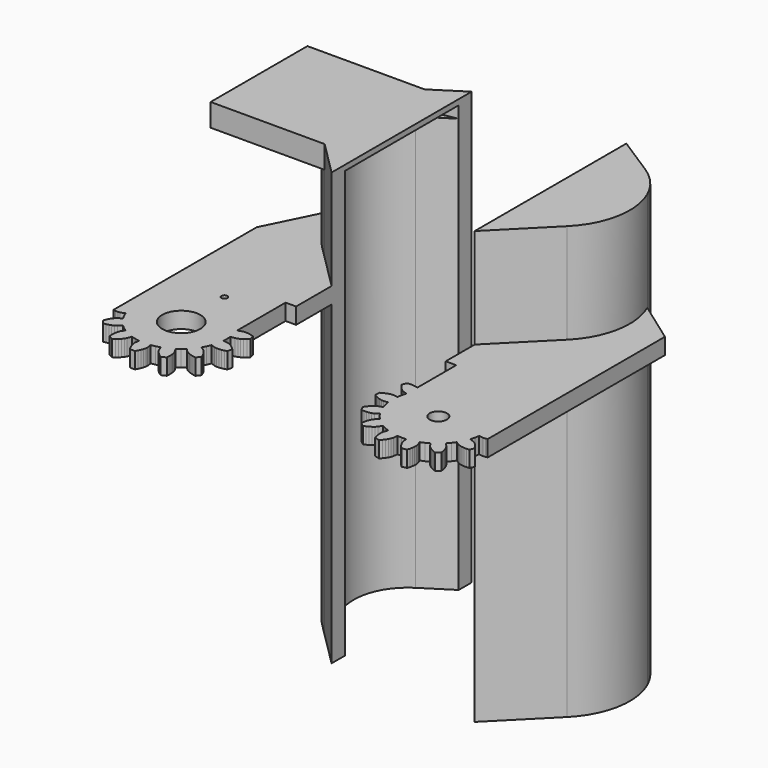
from build123d import *

# Parameters (mm, degrees)
F1_DEPTH  = 1.5
F0_R      = 1.6
F2_DEPTH  = 20
F3_DEPTH  = 60
F4_DEPTH  = 19
F5_DEPTH  = 16.8
F6_DEPTH  = 16.8
F7_DEPTH  = 15.8
F8_DEPTH  = 19
F9_DEPTH  = 15.8
F10_DEPTH = 1.5


# Not quite as in the source:
# - ends of sketch curves that miss each other by under 0.0002 mm in the source are joined


with BuildPart() as f1:
    # F0 (on Top) → F1 (new body, symmetric)
    with BuildSketch(Plane.XY):
        Polygon((-12.6828804, -37.9996929195), (-11.8884367355, -38.2222305677), (-11.8880267366, -38.2224279172), (-11.075543, -38.3664943195), (-11.1792258, -39.1773131195), (-11.1500412, -39.5862277195), (-11.049381, -40.0020257195), (-10.8967016, -40.4206431195), (-10.6978958, -40.8390065195), (-10.4565196, -41.2543727195), (-9.5434404, -41.2543727195), (-9.302115, -40.8390065195), (-9.1033092, -40.4206431195), (-8.950579, -40.0020257195), (-8.8499188, -39.5862277195), (-8.820785, -39.1773131195), (-8.9244678, -38.3664943195), (-8.1119840634, -38.2224279172), (-8.1115408, -38.2223493195), (-7.3171558, -37.9996929195), (-7.0589394, -38.7751549195), (-6.8550028, -39.1308311195), (-6.5838324, -39.4619201195), (-6.2647068, -39.7727145195), (-5.9041792, -40.0633667195), (-5.5066184, -40.3329369195), (-4.6838108, -39.9365445195), (-4.646549, -39.4578053195), (-4.6491144, -38.9947125195), (-4.693031, -38.5513555195), (-4.7828454, -38.1327635195), (-4.9339246, -37.7516365195), (-5.3789072, -37.0664715195), (-4.7096916266, -36.5840362135), (-4.709287, -36.5837445195), (-4.0899842, -36.0385589195), (-3.5209988, -36.6249941195), (-3.1831534, -36.8570993195), (-2.7948636, -37.0377695195), (-2.3725632, -37.1791713195), (-1.9218148, -37.2846829195), (-1.4464538, -37.3550663195), (-0.8770112, -36.6409453195), (-1.0512806, -36.1933973195), (-1.2544552, -35.7773199195), (-1.4865096, -35.3969041195), (-1.7489424, -35.0588555195), (-2.0504658, -34.7809287195), (-2.7488388, -34.3565455195), (-2.3551745142, -33.6315615111), (-2.3549356, -33.6311215195), (-2.0336002, -32.8714075195), (-1.2662154, -33.1527887195), (-0.86106, -33.2152727195), (-0.4331716, -33.2096847195), (0.0087884, -33.1539317195), (0.4607052, -33.0533223195), (0.9195562, -32.9104727195), (1.1227562, -32.0200757195), (0.7714742, -31.6924411195), (0.4079494, -31.4057259195), (0.033782, -31.1636639195), (-0.3494024, -30.9728083195), (-0.741426, -30.8533775195), (-1.5548356, -30.7739771195), (-1.5148031909, -29.9499745831), (-1.5147798, -29.9494931195), (-1.5548356, -29.1254663195), (-0.741426, -29.0460913195), (-0.3494024, -28.9266605195), (0.033782, -28.7358049195), (0.4079494, -28.4937683195), (0.7714742, -28.2070531195), (1.1227562, -27.8793931195), (0.9195562, -26.9889961195), (0.4607052, -26.8461465195), (0.0087884, -26.7455371195), (-0.4331716, -26.6898095195), (-0.86106, -26.6842215195), (-1.2662154, -26.7467055195), (-1.999996, -27.0157423195), (-1.999996, -15.8072914928), (-0.05, -15.8072914928), (-0.05, -8.999886363), (-7.8088611939, -1.2753778), (-20.002250767, -1.2753778), (-20.0087992, -33.1539317195), (-19.5667884, -33.2096847195), (-19.1389, -33.2152727195), (-18.7337954, -33.1527887195), (-17.9664106, -32.8714075195), (-17.6450069939, -33.6311141557), (-17.6448212, -33.6315533195), (-17.251172, -34.3565455195), (-17.9495196, -34.7809287195), (-18.2510684, -35.0588555195), (-18.5134504, -35.3969041195), (-18.745581, -35.7773199195), (-18.9487302, -36.1933973195), (-19.1229996, -36.6409453195), (-18.5535062, -37.3550663195), (-18.078196, -37.2846829195), (-17.6274476, -37.1791713195), (-17.2051218, -37.0377695195), (-16.8168066, -36.8570993195), (-16.479012, -36.6249941195), (-15.9100012, -36.0385589195), (-15.2906723648, -36.583686083), (-15.2903174, -36.5839985195), (-14.6211036, -37.0664715195), (-15.0660862, -37.7516365195), (-15.2171654, -38.1327635195), (-15.306929, -38.5513555195), (-15.3509218, -38.9947125195), (-15.3534618, -39.4578053195), (-15.3162, -39.9365445195), (-14.493367, -40.3329369195), (-14.0958062, -40.0633667195), (-13.735304, -39.7727145195), (-13.4161784, -39.4619201195), (-13.1449572, -39.1308311195), (-12.9410968, -38.7751549195), align=None)
        with BuildLine():
            ThreePointArc((-9.99998, -26.4247471195), (-7.5074285963, -27.4571957159), (-6.47498, -29.9497471195))
            ThreePointArc((-6.47498, -29.9497471195), (-12.4925314037, -32.4422985232), (-9.99998, -26.4247471195))
        make_face(mode=Mode.SUBTRACT)
        with BuildLine():
            ThreePointArc((-9.4549722, -19.9497471195), (-9.6146012888, -20.3351258307), (-9.99998, -20.4947549195))
            ThreePointArc((-9.99998, -20.4947549195), (-10.3853587112, -19.5643684084), (-9.4549722, -19.9497471195))
        make_face(mode=Mode.SUBTRACT)
        Polygon((-6.3914999282, -1.2753778), (-7.8088611939, -1.2753778), (-0.05, -8.999886363), (-0.05, -7.5888005143), align=None)
        Polygon((-8.4115295291, -0.6753778), (-7.8088611939, -1.2753778), (-6.3914999282, -1.2753778), (-6.9941682635, -0.6753778), align=None)
        with BuildLine():
            Line((-20.0019887813, 0), (-20.0021275162, -0.6753778))
            Line((-20.0021275162, -0.6753778), (-8.4115295291, -0.6753778))
            Line((-8.4115295291, -0.6753778), (-6.9941682635, -0.6753778))
            Line((-6.9941682635, -0.6753778), (-8.8192027426, 1.1415762748))
            ThreePointArc((-8.8192027426, 1.1415762748), (-11.5431807788, 5.203648739), (-12.5000003164, 10))
            Line((-12.5000003164, 10), (-15.0591228454, 10))
            Line((-15.0591228454, 10), (-20.0019887813, 0))
        make_face()
        with BuildLine():
            Line((-12.1022985118, 15.9820039061), (-15.0591228454, 10))
            Line((-15.0591228454, 10), (-12.5000003164, 10))
            ThreePointArc((-12.5000003164, 10), (-11.8911847625, 13.8535351113), (-10.1240431199, 17.331695494))
            Line((-10.1240431199, 17.331695494), (-12.1022985118, 15.9820039061))
        make_face()
        Polygon((-20.0021275162, -0.6753778), (-20.002250767, -1.2753778), (-7.8088611939, -1.2753778), (-8.4115295291, -0.6753778), align=None)
    extrude(amount=F1_DEPTH, both=True)



with BuildPart() as f1b:
    # F0 (on Top) → F1, piece 2 (new body, symmetric)
    with BuildSketch(Plane.XY):
        with BuildLine():
            Line((45.5568809356, -32.5242657195), (45.7794119864, -31.729845607))
            Line((45.7794119864, -31.729845607), (45.7796203111, -31.7294128346))
            Line((45.7796203111, -31.7294128346), (45.9237077356, -30.9169283195))
            Line((45.9237077356, -30.9169283195), (46.7345011356, -31.0206111195))
            Line((46.7345011356, -31.0206111195), (47.1434157356, -30.9914519195))
            Line((47.1434157356, -30.9914519195), (47.5068643356, -30.9034663195))
            Line((47.5068643356, -30.9034663195), (47.5068643356, 10.1083564))
            Line((47.5068643356, 10.1083564), (39.8461772472, 15.5849402666))
            ThreePointArc((39.8461772472, 15.5849402666), (40.7766908436, 7.6257287323), (37.0316684565, 0.541259019))
            Line((37.0316684565, 0.541259019), (27.5569297356, -8.9911811067))
            Line((27.5569297356, -8.9911811067), (27.5569297356, -15.6989350928))
            Line((27.5569297356, -15.6989350928), (29.5069257356, -15.6989350928))
            Line((29.5069257356, -15.6989350928), (29.5069257356, -24.6967985195))
            Line((29.5069257356, -24.6967985195), (29.3238933356, -24.6242561195))
            Line((29.3238933356, -24.6242561195), (28.9053267356, -24.5344163195))
            Line((28.9053267356, -24.5344163195), (28.4619443356, -24.4904997195))
            Line((28.4619443356, -24.4904997195), (27.9988769356, -24.4879343195))
            Line((27.9988769356, -24.4879343195), (27.5201123356, -24.5252215195))
            Line((27.5201123356, -24.5252215195), (27.1237453356, -25.3480037195))
            Line((27.1237453356, -25.3480037195), (27.3933155356, -25.7455645195))
            Line((27.3933155356, -25.7455645195), (27.6839931356, -26.1060921195))
            Line((27.6839931356, -26.1060921195), (27.9947367356, -26.4252177195))
            Line((27.9947367356, -26.4252177195), (28.3259019356, -26.6964135195))
            Line((28.3259019356, -26.6964135195), (28.6815781356, -26.9003247195))
            Line((28.6815781356, -26.9003247195), (29.4569385356, -27.1585411195))
            Line((29.4569385356, -27.1585411195), (29.2345090358, -27.9529612023))
            Line((29.2345090358, -27.9529612023), (29.2343837356, -27.9534087195))
            Line((29.2343837356, -27.9534087195), (29.0901625356, -28.7658785195))
            Line((29.0901625356, -28.7658785195), (28.2793183356, -28.6621957195))
            Line((28.2793183356, -28.6621957195), (27.8704545356, -28.6913041195))
            Line((27.8704545356, -28.6913041195), (27.4546819356, -28.7919643195))
            Line((27.4546819356, -28.7919643195), (27.0360137356, -28.9447199195))
            Line((27.0360137356, -28.9447199195), (26.6177011356, -29.1435003195))
            Line((26.6177011356, -29.1435003195), (26.2023095356, -29.3848257195))
            Line((26.2023095356, -29.3848257195), (26.2023095356, -30.2979303195))
            Line((26.2023095356, -30.2979303195), (26.6177011356, -30.5392811195))
            Line((26.6177011356, -30.5392811195), (27.0360137356, -30.7380869195))
            Line((27.0360137356, -30.7380869195), (27.4546819356, -30.8907917195))
            Line((27.4546819356, -30.8907917195), (27.8704545356, -30.9914519195))
            Line((27.8704545356, -30.9914519195), (28.2793183356, -31.0206111195))
            Line((28.2793183356, -31.0206111195), (29.0901625356, -30.9169283195))
            Line((29.0901625356, -30.9169283195), (29.2343007326, -31.7294128446))
            Line((29.2343007326, -31.7294128446), (29.2343837356, -31.7298807195))
            Line((29.2343837356, -31.7298807195), (29.4569385356, -32.5242657195))
            Line((29.4569385356, -32.5242657195), (28.6815781356, -32.7824821195))
            Line((28.6815781356, -32.7824821195), (28.3259019356, -32.9863679195))
            Line((28.3259019356, -32.9863679195), (27.9947367356, -33.2575891195))
            Line((27.9947367356, -33.2575891195), (27.6839931356, -33.5766893195))
            Line((27.6839931356, -33.5766893195), (27.3933155356, -33.9371915195))
            Line((27.3933155356, -33.9371915195), (27.1237453356, -34.3347523195))
            Line((27.1237453356, -34.3347523195), (27.5201123356, -35.1575853195))
            Line((27.5201123356, -35.1575853195), (27.9988769356, -35.1948725195))
            Line((27.9988769356, -35.1948725195), (28.4619443356, -35.1923071195))
            Line((28.4619443356, -35.1923071195), (28.9053267356, -35.1483397195))
            Line((28.9053267356, -35.1483397195), (29.3238933356, -35.0585507195))
            Line((29.3238933356, -35.0585507195), (29.7050457356, -34.9074715195))
            Line((29.7050457356, -34.9074715195), (30.3902107356, -34.4624889195))
            Line((30.3902107356, -34.4624889195), (30.8726460484, -35.1317298871))
            Line((30.8726460484, -35.1317298871), (30.8729377356, -35.1321345195))
            Line((30.8729377356, -35.1321345195), (31.4180979356, -35.7513865195))
            Line((31.4180979356, -35.7513865195), (30.8316881356, -36.3203973195))
            Line((30.8316881356, -36.3203973195), (30.5995829356, -36.6582173195))
            Line((30.5995829356, -36.6582173195), (30.4189127356, -37.0465071195))
            Line((30.4189127356, -37.0465071195), (30.2775109356, -37.4688583195))
            Line((30.2775109356, -37.4688583195), (30.1719993356, -37.9196067195))
            Line((30.1719993356, -37.9196067195), (30.1016159356, -38.3949169195))
            Line((30.1016159356, -38.3949169195), (30.8157369356, -38.9643849195))
            Line((30.8157369356, -38.9643849195), (31.2632849356, -38.7901155195))
            Line((31.2632849356, -38.7901155195), (31.6793623356, -38.5869663195))
            Line((31.6793623356, -38.5869663195), (32.0597527356, -38.3548611195))
            Line((32.0597527356, -38.3548611195), (32.3978267356, -38.0924537195))
            Line((32.3978267356, -38.0924537195), (32.6757535356, -37.7909049195))
            Line((32.6757535356, -37.7909049195), (33.1001367356, -37.0925827195))
            Line((33.1001367356, -37.0925827195), (33.8251420267, -37.4861824058))
            Line((33.8251420267, -37.4861824058), (33.8255607356, -37.4864097195))
            Line((33.8255607356, -37.4864097195), (34.5852747356, -37.8077959195))
            Line((34.5852747356, -37.8077959195), (34.3038935356, -38.5752061195))
            Line((34.3038935356, -38.5752061195), (34.2414095356, -38.9803107195))
            Line((34.2414095356, -38.9803107195), (34.2469975356, -39.4081737195))
            Line((34.2469975356, -39.4081737195), (34.3027505356, -39.8501845195))
            Line((34.3027505356, -39.8501845195), (34.4033599356, -40.3021267195))
            Line((34.4033599356, -40.3021267195), (34.5461841356, -40.7609777195))
            Line((34.5461841356, -40.7609777195), (35.4366065356, -40.9641777195))
            Line((35.4366065356, -40.9641777195), (35.7642411356, -40.6128957195))
            Line((35.7642411356, -40.6128957195), (36.0509563356, -40.2493201195))
            Line((36.0509563356, -40.2493201195), (36.2929929356, -39.8751781195))
            Line((36.2929929356, -39.8751781195), (36.4838739356, -39.4919429195))
            Line((36.4838739356, -39.4919429195), (36.6033047356, -39.0999955195))
            Line((36.6033047356, -39.0999955195), (36.6826797356, -38.2865605195))
            Line((36.6826797356, -38.2865605195), (37.5067076121, -38.3265941598))
            Line((37.5067076121, -38.3265941598), (37.5071637356, -38.3266163195))
            Line((37.5071637356, -38.3266163195), (38.3311651356, -38.2865605195))
            Line((38.3311651356, -38.2865605195), (38.4105909356, -39.0999955195))
            Line((38.4105909356, -39.0999955195), (38.5299963356, -39.4919429195))
            Line((38.5299963356, -39.4919429195), (38.7208773356, -39.8751781195))
            Line((38.7208773356, -39.8751781195), (38.9629139356, -40.2493201195))
            Line((38.9629139356, -40.2493201195), (39.2496291356, -40.6128957195))
            Line((39.2496291356, -40.6128957195), (39.5772891356, -40.9641777195))
            Line((39.5772891356, -40.9641777195), (40.4676861356, -40.7609777195))
            Line((40.4676861356, -40.7609777195), (40.6105103356, -40.3021267195))
            Line((40.6105103356, -40.3021267195), (40.7111451356, -39.8501845195))
            Line((40.7111451356, -39.8501845195), (40.7668727356, -39.4081737195))
            Line((40.7668727356, -39.4081737195), (40.7724607356, -38.9803107195))
            Line((40.7724607356, -38.9803107195), (40.7099767356, -38.5752061195))
            Line((40.7099767356, -38.5752061195), (40.4285955356, -37.8077959195))
            Line((40.4285955356, -37.8077959195), (41.1883021717, -37.4863923134))
            Line((41.1883021717, -37.4863923134), (41.1887413356, -37.4862065195))
            Line((41.1887413356, -37.4862065195), (41.9137335356, -37.0925827195))
            Line((41.9137335356, -37.0925827195), (42.3381421356, -37.7909049195))
            Line((42.3381421356, -37.7909049195), (42.6160435356, -38.0924537195))
            Line((42.6160435356, -38.0924537195), (42.9541175356, -38.3548611195))
            Line((42.9541175356, -38.3548611195), (43.3345079356, -38.5869663195))
            Line((43.3345079356, -38.5869663195), (43.7505853356, -38.7901155195))
            Line((43.7505853356, -38.7901155195), (44.1981333356, -38.9643849195))
            Line((44.1981333356, -38.9643849195), (44.9122543356, -38.3949169195))
            Line((44.9122543356, -38.3949169195), (44.8418709356, -37.9196067195))
            Line((44.8418709356, -37.9196067195), (44.7363593356, -37.4688583195))
            Line((44.7363593356, -37.4688583195), (44.5949575356, -37.0465071195))
            Line((44.5949575356, -37.0465071195), (44.4142873356, -36.6582173195))
            Line((44.4142873356, -36.6582173195), (44.1821821356, -36.3203973195))
            Line((44.1821821356, -36.3203973195), (43.5957723356, -35.7513865195))
            Line((43.5957723356, -35.7513865195), (44.1408615089, -35.1320720054))
            Line((44.1408615089, -35.1320720054), (44.1411865356, -35.1317027195))
            Line((44.1411865356, -35.1317027195), (44.6236595356, -34.4624889195))
            Line((44.6236595356, -34.4624889195), (45.3088245356, -34.9074715195))
            Line((45.3088245356, -34.9074715195), (45.6899769356, -35.0585507195))
            Line((45.6899769356, -35.0585507195), (46.1085435356, -35.1483397195))
            Line((46.1085435356, -35.1483397195), (46.5519259356, -35.1923071195))
            Line((46.5519259356, -35.1923071195), (47.0149933356, -35.1948725195))
            Line((47.0149933356, -35.1948725195), (47.4937325356, -35.1575853195))
            Line((47.4937325356, -35.1575853195), (47.8901249356, -34.3347523195))
            Line((47.8901249356, -34.3347523195), (47.6205547356, -33.9371915195))
            Line((47.6205547356, -33.9371915195), (47.3299025356, -33.5766893195))
            Line((47.3299025356, -33.5766893195), (47.0191335356, -33.2575891195))
            Line((47.0191335356, -33.2575891195), (46.6880191356, -32.9863679195))
            Line((46.6880191356, -32.9863679195), (46.3323429356, -32.7824821195))
            Line((46.3323429356, -32.7824821195), (45.5568809356, -32.5242657195))
        make_face()
        with Locations((37.5069097356, -29.8413907195)):
            Circle(F0_R, mode=Mode.SUBTRACT)
    extrude(amount=F1_DEPTH, both=True)



with BuildPart() as f2:
    # F0 (on Top) → F2 (new body)
    with BuildSketch(Plane.XY):
        with BuildLine():
            Line((-8.8192027426, 1.1415762748), (-6.9941682635, -0.6753778))
            Line((-6.9941682635, -0.6753778), (-0.05, -4.5405198881))
            Line((-0.05, -4.5405198881), (-7.28327834, 3.1477115777))
            ThreePointArc((-7.28327834, 3.1477115777), (-9.9219987158, 11.2465718924), (-5.3618740808, 18.4409896542))
            Line((-5.3618740808, 18.4409896542), (-0.05, 21.8151911543))
            Line((-0.05, 21.8151911543), (-6.7420944452, 20.5258809799))
            ThreePointArc((-6.7420944452, 20.5258809799), (-8.5829688524, 19.0874998536), (-10.1240431199, 17.331695494))
            ThreePointArc((-10.1240431199, 17.331695494), (-11.8911847625, 13.8535351113), (-12.5000003164, 10))
            ThreePointArc((-12.5000003164, 10), (-11.5431807788, 5.203648739), (-8.8192027426, 1.1415762748))
        make_face()
        Polygon((-5.8053634872, 21.1258809799), (-6.7420944452, 20.5258809799), (-0.05, 21.8151911543), (-0.05, 22.999886363), (-0.05, 24.8123376548), align=None)
        Polygon((-6.9941682635, -0.6753778), (-6.3914999282, -1.2753778), (-0.05, -7.5888005143), (-0.05, -5.999886363), (-0.05, -4.5405198881), align=None)
        with BuildLine():
            Line((-7.28327834, 3.1477115777), (-0.05, -4.5405198881))
            Line((-0.05, -4.5405198881), (-0.05, 21.8151911543))
            Line((-0.05, 21.8151911543), (-5.3618740808, 18.4409896542))
            ThreePointArc((-5.3618740808, 18.4409896542), (-9.9219987158, 11.2465718924), (-7.28327834, 3.1477115777))
        make_face()
        with BuildLine():
            ThreePointArc((-17.0059758203, 20.5258809799), (-19.2368888885, 15.4716989952), (-19.9999346, 10))
            Line((-19.9999346, 10), (-15.0591228454, 10))
            Line((-15.0591228454, 10), (-12.1022985118, 15.9820039061))
            Line((-12.1022985118, 15.9820039061), (-10.1240431199, 17.331695494))
            ThreePointArc((-10.1240431199, 17.331695494), (-8.5829688524, 19.0874998536), (-6.7420944452, 20.5258809799))
            Line((-6.7420944452, 20.5258809799), (-17.0059758203, 20.5258809799))
        make_face()
        with BuildLine():
            Line((-27.5000003164, 10), (-19.9999346, 10))
            ThreePointArc((-19.9999346, 10), (-19.2368888885, 15.4716989952), (-17.0059758203, 20.5258809799))
            Line((-17.0059758203, 20.5258809799), (-27.5000003164, 20.5258809799))
            Line((-27.5000003164, 20.5258809799), (-27.5000003164, 10))
        make_face()
        Polygon((-27.5000003164, -0.6753778), (-20.0021275162, -0.6753778), (-20.0019887813, 0), (-19.9999346, 10), (-27.5000003164, 10), align=None)
        Polygon((-19.9999346, 10), (-20.0019887813, 0), (-15.0591228454, 10), align=None)
        with BuildLine():
            Line((-20.0019887813, 0), (-20.0021275162, -0.6753778))
            Line((-20.0021275162, -0.6753778), (-8.4115295291, -0.6753778))
            Line((-8.4115295291, -0.6753778), (-6.9941682635, -0.6753778))
            Line((-6.9941682635, -0.6753778), (-8.8192027426, 1.1415762748))
            ThreePointArc((-8.8192027426, 1.1415762748), (-11.5431807788, 5.203648739), (-12.5000003164, 10))
            Line((-12.5000003164, 10), (-15.0591228454, 10))
            Line((-15.0591228454, 10), (-20.0019887813, 0))
        make_face()
        with BuildLine():
            Line((-12.1022985118, 15.9820039061), (-15.0591228454, 10))
            Line((-15.0591228454, 10), (-12.5000003164, 10))
            ThreePointArc((-12.5000003164, 10), (-11.8911847625, 13.8535351113), (-10.1240431199, 17.331695494))
            Line((-10.1240431199, 17.331695494), (-12.1022985118, 15.9820039061))
        make_face()
        with BuildLine():
            ThreePointArc((-16.6196316573, 21.1258809799), (-16.8154800574, 20.82760428), (-17.0059758203, 20.5258809799))
            Line((-17.0059758203, 20.5258809799), (-6.7420944452, 20.5258809799))
            Line((-6.7420944452, 20.5258809799), (-5.8053634872, 21.1258809799))
            Line((-5.8053634872, 21.1258809799), (-16.6196316573, 21.1258809799))
        make_face()
        with BuildLine():
            Line((-27.5000003164, 20.5258809799), (-17.0059758203, 20.5258809799))
            ThreePointArc((-17.0059758203, 20.5258809799), (-16.8154800574, 20.82760428), (-16.6196316573, 21.1258809799))
            Line((-16.6196316573, 21.1258809799), (-27.5000003164, 21.1258809799))
            Line((-27.5000003164, 21.1258809799), (-27.5000003164, 20.5258809799))
        make_face()
        Polygon((-8.4115295291, -0.6753778), (-7.8088611939, -1.2753778), (-6.3914999282, -1.2753778), (-6.9941682635, -0.6753778), align=None)
        Polygon((-20.0021275162, -0.6753778), (-20.002250767, -1.2753778), (-7.8088611939, -1.2753778), (-8.4115295291, -0.6753778), align=None)
        Polygon((-27.5000003164, -1.2753778), (-20.002250767, -1.2753778), (-20.0021275162, -0.6753778), (-27.5000003164, -0.6753778), align=None)
    extrude(amount=F2_DEPTH)


with BuildPart() as f2b:
    # F0 (on Top) → F2, piece 2 (new body)
    with BuildSketch(Plane.XY):
        with BuildLine():
            Line((33.4049912244, 19.3934450196), (27.5569297356, 23.108242763))
            Line((27.5569297356, 23.108242763), (27.5569297356, 21.9235484419))
            Line((27.5569297356, 21.9235484419), (32.868804218, 18.5493466866))
            ThreePointArc((32.868804218, 18.5493466866), (37.4289291947, 11.3549283858), (34.7902086212, 3.2560674644))
            Line((34.7902086212, 3.2560674644), (27.5569297356, -4.4321645815))
            Line((27.5569297356, -4.4321645815), (27.5569297356, -5.891529963))
            Line((27.5569297356, -5.891529963), (35.5185359096, 2.5708391355))
            ThreePointArc((35.5185359096, 2.5708391355), (38.421128323, 11.4795854816), (33.4049912244, 19.3934450196))
        make_face()
        with BuildLine():
            ThreePointArc((37.0316684565, 0.541259019), (40.7766908436, 7.6257287323), (39.8461772472, 15.5849402666))
            ThreePointArc((39.8461772472, 15.5849402666), (37.7499815665, 18.9020978784), (34.788391552, 21.4763075705))
            Line((34.788391552, 21.4763075705), (27.5569297356, 26.108242763))
            Line((27.5569297356, 26.108242763), (27.5569297356, 23.108242763))
            Line((27.5569297356, 23.108242763), (33.4049912244, 19.3934450196))
            ThreePointArc((33.4049912244, 19.3934450196), (38.421128323, 11.4795854816), (35.5185359096, 2.5708391355))
            Line((35.5185359096, 2.5708391355), (27.5569297356, -5.891529963))
            Line((27.5569297356, -5.891529963), (27.5569297356, -8.9911811067))
            Line((27.5569297356, -8.9911811067), (37.0316684565, 0.541259019))
        make_face()
        with BuildLine():
            Line((32.868804218, 18.5493466866), (27.5569297356, 21.9235484419))
            Line((27.5569297356, 21.9235484419), (27.5569297356, -4.4321645815))
            Line((27.5569297356, -4.4321645815), (34.7902086212, 3.2560674644))
            ThreePointArc((34.7902086212, 3.2560674644), (37.4289291947, 11.3549283858), (32.868804218, 18.5493466866))
        make_face()
    extrude(amount=F2_DEPTH)


with BuildPart() as f1_1:
    add(f1.part)

    add(f2.part)  # F3 merges F2
    # F0 (on Top) → F3 (join)
    with BuildSketch(Plane.XY):
        with BuildLine():
            Line((-8.8192027426, 1.1415762748), (-6.9941682635, -0.6753778))
            Line((-6.9941682635, -0.6753778), (-0.05, -4.5405198881))
            Line((-0.05, -4.5405198881), (-7.28327834, 3.1477115777))
            ThreePointArc((-7.28327834, 3.1477115777), (-9.9219987158, 11.2465718924), (-5.3618740808, 18.4409896542))
            Line((-5.3618740808, 18.4409896542), (-0.05, 21.8151911543))
            Line((-0.05, 21.8151911543), (-6.7420944452, 20.5258809799))
            ThreePointArc((-6.7420944452, 20.5258809799), (-8.5829688524, 19.0874998536), (-10.1240431199, 17.331695494))
            ThreePointArc((-10.1240431199, 17.331695494), (-11.8911847625, 13.8535351113), (-12.5000003164, 10))
            ThreePointArc((-12.5000003164, 10), (-11.5431807788, 5.203648739), (-8.8192027426, 1.1415762748))
        make_face()
        Polygon((-6.9941682635, -0.6753778), (-6.3914999282, -1.2753778), (-0.05, -7.5888005143), (-0.05, -5.999886363), (-0.05, -4.5405198881), align=None)
        Polygon((-5.8053634872, 21.1258809799), (-6.7420944452, 20.5258809799), (-0.05, 21.8151911543), (-0.05, 22.999886363), (-0.05, 24.8123376548), align=None)
    extrude(amount=-F3_DEPTH)


with BuildPart() as f1b_1:
    add(f1b.part)

    add(f2b.part)  # F3#2 merges F2b
    # F0 (on Top) → F3, piece 2 (join)
    with BuildSketch(Plane.XY):
        with BuildLine():
            Line((33.4049912244, 19.3934450196), (27.5569297356, 23.108242763))
            Line((27.5569297356, 23.108242763), (27.5569297356, 21.9235484419))
            Line((27.5569297356, 21.9235484419), (32.868804218, 18.5493466866))
            ThreePointArc((32.868804218, 18.5493466866), (37.4289291947, 11.3549283858), (34.7902086212, 3.2560674644))
            Line((34.7902086212, 3.2560674644), (27.5569297356, -4.4321645815))
            Line((27.5569297356, -4.4321645815), (27.5569297356, -5.891529963))
            Line((27.5569297356, -5.891529963), (35.5185359096, 2.5708391355))
            ThreePointArc((35.5185359096, 2.5708391355), (38.421128323, 11.4795854816), (33.4049912244, 19.3934450196))
        make_face()
        with BuildLine():
            ThreePointArc((37.0316684565, 0.541259019), (40.7766908436, 7.6257287323), (39.8461772472, 15.5849402666))
            ThreePointArc((39.8461772472, 15.5849402666), (37.7499815665, 18.9020978784), (34.788391552, 21.4763075705))
            Line((34.788391552, 21.4763075705), (27.5569297356, 26.108242763))
            Line((27.5569297356, 26.108242763), (27.5569297356, 23.108242763))
            Line((27.5569297356, 23.108242763), (33.4049912244, 19.3934450196))
            ThreePointArc((33.4049912244, 19.3934450196), (38.421128323, 11.4795854816), (35.5185359096, 2.5708391355))
            Line((35.5185359096, 2.5708391355), (27.5569297356, -5.891529963))
            Line((27.5569297356, -5.891529963), (27.5569297356, -8.9911811067))
            Line((27.5569297356, -8.9911811067), (37.0316684565, 0.541259019))
        make_face()
    extrude(amount=-F3_DEPTH)


with BuildPart() as f4_tool:
    # F0 (on Top) → F4 (new body)
    with BuildSketch(Plane.XY):
        with BuildLine():
            Line((-8.8192027426, 1.1415762748), (-6.9941682635, -0.6753778))
            Line((-6.9941682635, -0.6753778), (-0.05, -4.5405198881))
            Line((-0.05, -4.5405198881), (-7.28327834, 3.1477115777))
            ThreePointArc((-7.28327834, 3.1477115777), (-9.9219987158, 11.2465718924), (-5.3618740808, 18.4409896542))
            Line((-5.3618740808, 18.4409896542), (-0.05, 21.8151911543))
            Line((-0.05, 21.8151911543), (-6.7420944452, 20.5258809799))
            ThreePointArc((-6.7420944452, 20.5258809799), (-8.5829688524, 19.0874998536), (-10.1240431199, 17.331695494))
            ThreePointArc((-10.1240431199, 17.331695494), (-11.8911847625, 13.8535351113), (-12.5000003164, 10))
            ThreePointArc((-12.5000003164, 10), (-11.5431807788, 5.203648739), (-8.8192027426, 1.1415762748))
        make_face()
        with BuildLine():
            Line((-7.28327834, 3.1477115777), (-0.05, -4.5405198881))
            Line((-0.05, -4.5405198881), (-0.05, 21.8151911543))
            Line((-0.05, 21.8151911543), (-5.3618740808, 18.4409896542))
            ThreePointArc((-5.3618740808, 18.4409896542), (-9.9219987158, 11.2465718924), (-7.28327834, 3.1477115777))
        make_face()
        with BuildLine():
            Line((32.868804218, 18.5493466866), (27.5569297356, 21.9235484419))
            Line((27.5569297356, 21.9235484419), (27.5569297356, -4.4321645815))
            Line((27.5569297356, -4.4321645815), (34.7902086212, 3.2560674644))
            ThreePointArc((34.7902086212, 3.2560674644), (37.4289291947, 11.3549283858), (32.868804218, 18.5493466866))
        make_face()
        Polygon((-27.5000003164, -0.6753778), (-20.0021275162, -0.6753778), (-20.0019887813, 0), (-19.9999346, 10), (-27.5000003164, 10), align=None)
        Polygon((-19.9999346, 10), (-20.0019887813, 0), (-15.0591228454, 10), align=None)
        with BuildLine():
            Line((-20.0019887813, 0), (-20.0021275162, -0.6753778))
            Line((-20.0021275162, -0.6753778), (-8.4115295291, -0.6753778))
            Line((-8.4115295291, -0.6753778), (-6.9941682635, -0.6753778))
            Line((-6.9941682635, -0.6753778), (-8.8192027426, 1.1415762748))
            ThreePointArc((-8.8192027426, 1.1415762748), (-11.5431807788, 5.203648739), (-12.5000003164, 10))
            Line((-12.5000003164, 10), (-15.0591228454, 10))
            Line((-15.0591228454, 10), (-20.0019887813, 0))
        make_face()
        with BuildLine():
            Line((-12.1022985118, 15.9820039061), (-15.0591228454, 10))
            Line((-15.0591228454, 10), (-12.5000003164, 10))
            ThreePointArc((-12.5000003164, 10), (-11.8911847625, 13.8535351113), (-10.1240431199, 17.331695494))
            Line((-10.1240431199, 17.331695494), (-12.1022985118, 15.9820039061))
        make_face()
        with BuildLine():
            ThreePointArc((-17.0059758203, 20.5258809799), (-19.2368888885, 15.4716989952), (-19.9999346, 10))
            Line((-19.9999346, 10), (-15.0591228454, 10))
            Line((-15.0591228454, 10), (-12.1022985118, 15.9820039061))
            Line((-12.1022985118, 15.9820039061), (-10.1240431199, 17.331695494))
            ThreePointArc((-10.1240431199, 17.331695494), (-8.5829688524, 19.0874998536), (-6.7420944452, 20.5258809799))
            Line((-6.7420944452, 20.5258809799), (-17.0059758203, 20.5258809799))
        make_face()
        with BuildLine():
            Line((-27.5000003164, 10), (-19.9999346, 10))
            ThreePointArc((-19.9999346, 10), (-19.2368888885, 15.4716989952), (-17.0059758203, 20.5258809799))
            Line((-17.0059758203, 20.5258809799), (-27.5000003164, 20.5258809799))
            Line((-27.5000003164, 20.5258809799), (-27.5000003164, 10))
        make_face()
        Polygon((-20.0021275162, -0.6753778), (-20.002250767, -1.2753778), (-7.8088611939, -1.2753778), (-8.4115295291, -0.6753778), align=None)
        Polygon((-8.4115295291, -0.6753778), (-7.8088611939, -1.2753778), (-6.3914999282, -1.2753778), (-6.9941682635, -0.6753778), align=None)
        with BuildLine():
            ThreePointArc((-16.6196316573, 21.1258809799), (-16.8154800574, 20.82760428), (-17.0059758203, 20.5258809799))
            Line((-17.0059758203, 20.5258809799), (-6.7420944452, 20.5258809799))
            Line((-6.7420944452, 20.5258809799), (-5.8053634872, 21.1258809799))
            Line((-5.8053634872, 21.1258809799), (-16.6196316573, 21.1258809799))
        make_face()
        Polygon((-27.5000003164, -1.2753778), (-20.002250767, -1.2753778), (-20.0021275162, -0.6753778), (-27.5000003164, -0.6753778), align=None)
        with BuildLine():
            Line((-27.5000003164, 20.5258809799), (-17.0059758203, 20.5258809799))
            ThreePointArc((-17.0059758203, 20.5258809799), (-16.8154800574, 20.82760428), (-16.6196316573, 21.1258809799))
            Line((-16.6196316573, 21.1258809799), (-27.5000003164, 21.1258809799))
            Line((-27.5000003164, 21.1258809799), (-27.5000003164, 20.5258809799))
        make_face()
    extrude(amount=F4_DEPTH)


with BuildPart() as f1_2:
    add(f1_1.part)

    # F4: cut by f4_tool
    add(f4_tool.part, mode=Mode.SUBTRACT)

    # F0 (on Top) → F5 (join)
    with BuildSketch(Plane.XY):
        with BuildLine():
            Line((-8.8192027426, 1.1415762748), (-6.9941682635, -0.6753778))
            Line((-6.9941682635, -0.6753778), (-0.05, -4.5405198881))
            Line((-0.05, -4.5405198881), (-7.28327834, 3.1477115777))
            ThreePointArc((-7.28327834, 3.1477115777), (-9.9219987158, 11.2465718924), (-5.3618740808, 18.4409896542))
            Line((-5.3618740808, 18.4409896542), (-0.05, 21.8151911543))
            Line((-0.05, 21.8151911543), (-6.7420944452, 20.5258809799))
            ThreePointArc((-6.7420944452, 20.5258809799), (-8.5829688524, 19.0874998536), (-10.1240431199, 17.331695494))
            ThreePointArc((-10.1240431199, 17.331695494), (-11.8911847625, 13.8535351113), (-12.5000003164, 10))
            ThreePointArc((-12.5000003164, 10), (-11.5431807788, 5.203648739), (-8.8192027426, 1.1415762748))
        make_face()
    extrude(amount=F5_DEPTH)

    # F0 (on Top) → F6 (join)
    with BuildSketch(Plane.XY):
        with BuildLine():
            Line((-20.0019887813, 0), (-20.0021275162, -0.6753778))
            Line((-20.0021275162, -0.6753778), (-8.4115295291, -0.6753778))
            Line((-8.4115295291, -0.6753778), (-6.9941682635, -0.6753778))
            Line((-6.9941682635, -0.6753778), (-8.8192027426, 1.1415762748))
            ThreePointArc((-8.8192027426, 1.1415762748), (-11.5431807788, 5.203648739), (-12.5000003164, 10))
            Line((-12.5000003164, 10), (-15.0591228454, 10))
            Line((-15.0591228454, 10), (-20.0019887813, 0))
        make_face()
        Polygon((-19.9999346, 10), (-20.0019887813, 0), (-15.0591228454, 10), align=None)
        with BuildLine():
            ThreePointArc((-17.0059758203, 20.5258809799), (-19.2368888885, 15.4716989952), (-19.9999346, 10))
            Line((-19.9999346, 10), (-15.0591228454, 10))
            Line((-15.0591228454, 10), (-12.1022985118, 15.9820039061))
            Line((-12.1022985118, 15.9820039061), (-10.1240431199, 17.331695494))
            ThreePointArc((-10.1240431199, 17.331695494), (-8.5829688524, 19.0874998536), (-6.7420944452, 20.5258809799))
            Line((-6.7420944452, 20.5258809799), (-17.0059758203, 20.5258809799))
        make_face()
        with BuildLine():
            Line((-12.1022985118, 15.9820039061), (-15.0591228454, 10))
            Line((-15.0591228454, 10), (-12.5000003164, 10))
            ThreePointArc((-12.5000003164, 10), (-11.8911847625, 13.8535351113), (-10.1240431199, 17.331695494))
            Line((-10.1240431199, 17.331695494), (-12.1022985118, 15.9820039061))
        make_face()
    extrude(amount=F6_DEPTH)

    # F0 (on Top) → F7 (cut)
    with BuildSketch(Plane.XY):
        with BuildLine():
            Line((-20.0019887813, 0), (-20.0021275162, -0.6753778))
            Line((-20.0021275162, -0.6753778), (-8.4115295291, -0.6753778))
            Line((-8.4115295291, -0.6753778), (-6.9941682635, -0.6753778))
            Line((-6.9941682635, -0.6753778), (-8.8192027426, 1.1415762748))
            ThreePointArc((-8.8192027426, 1.1415762748), (-11.5431807788, 5.203648739), (-12.5000003164, 10))
            Line((-12.5000003164, 10), (-15.0591228454, 10))
            Line((-15.0591228454, 10), (-20.0019887813, 0))
        make_face()
        with BuildLine():
            Line((-12.1022985118, 15.9820039061), (-15.0591228454, 10))
            Line((-15.0591228454, 10), (-12.5000003164, 10))
            ThreePointArc((-12.5000003164, 10), (-11.8911847625, 13.8535351113), (-10.1240431199, 17.331695494))
            Line((-10.1240431199, 17.331695494), (-12.1022985118, 15.9820039061))
        make_face()
        Polygon((-19.9999346, 10), (-20.0019887813, 0), (-15.0591228454, 10), align=None)
        with BuildLine():
            ThreePointArc((-17.0059758203, 20.5258809799), (-19.2368888885, 15.4716989952), (-19.9999346, 10))
            Line((-19.9999346, 10), (-15.0591228454, 10))
            Line((-15.0591228454, 10), (-12.1022985118, 15.9820039061))
            Line((-12.1022985118, 15.9820039061), (-10.1240431199, 17.331695494))
            ThreePointArc((-10.1240431199, 17.331695494), (-8.5829688524, 19.0874998536), (-6.7420944452, 20.5258809799))
            Line((-6.7420944452, 20.5258809799), (-17.0059758203, 20.5258809799))
        make_face()
    extrude(amount=F7_DEPTH, mode=Mode.SUBTRACT)

    # F0 (on Top) → F8 (join)
    with BuildSketch(Plane.XY):
        Polygon((-8.4115295291, -0.6753778), (-7.8088611939, -1.2753778), (-6.3914999282, -1.2753778), (-6.9941682635, -0.6753778), align=None)
        Polygon((-20.0021275162, -0.6753778), (-20.002250767, -1.2753778), (-7.8088611939, -1.2753778), (-8.4115295291, -0.6753778), align=None)
        Polygon((-27.5000003164, -1.2753778), (-20.002250767, -1.2753778), (-20.0021275162, -0.6753778), (-27.5000003164, -0.6753778), align=None)
        with BuildLine():
            ThreePointArc((-16.6196316573, 21.1258809799), (-16.8154800574, 20.82760428), (-17.0059758203, 20.5258809799))
            Line((-17.0059758203, 20.5258809799), (-6.7420944452, 20.5258809799))
            Line((-6.7420944452, 20.5258809799), (-5.8053634872, 21.1258809799))
            Line((-5.8053634872, 21.1258809799), (-16.6196316573, 21.1258809799))
        make_face()
        with BuildLine():
            Line((-27.5000003164, 20.5258809799), (-17.0059758203, 20.5258809799))
            ThreePointArc((-17.0059758203, 20.5258809799), (-16.8154800574, 20.82760428), (-16.6196316573, 21.1258809799))
            Line((-16.6196316573, 21.1258809799), (-27.5000003164, 21.1258809799))
            Line((-27.5000003164, 21.1258809799), (-27.5000003164, 20.5258809799))
        make_face()
    extrude(amount=F8_DEPTH)

    # F0 (on Top) → F9 (cut)
    with BuildSketch(Plane.XY):
        Polygon((-8.4115295291, -0.6753778), (-7.8088611939, -1.2753778), (-6.3914999282, -1.2753778), (-6.9941682635, -0.6753778), align=None)
        Polygon((-20.0021275162, -0.6753778), (-20.002250767, -1.2753778), (-7.8088611939, -1.2753778), (-8.4115295291, -0.6753778), align=None)
        Polygon((-27.5000003164, -1.2753778), (-20.002250767, -1.2753778), (-20.0021275162, -0.6753778), (-27.5000003164, -0.6753778), align=None)
        with BuildLine():
            ThreePointArc((-16.6196316573, 21.1258809799), (-16.8154800574, 20.82760428), (-17.0059758203, 20.5258809799))
            Line((-17.0059758203, 20.5258809799), (-6.7420944452, 20.5258809799))
            Line((-6.7420944452, 20.5258809799), (-5.8053634872, 21.1258809799))
            Line((-5.8053634872, 21.1258809799), (-16.6196316573, 21.1258809799))
        make_face()
        with BuildLine():
            Line((-27.5000003164, 20.5258809799), (-17.0059758203, 20.5258809799))
            ThreePointArc((-17.0059758203, 20.5258809799), (-16.8154800574, 20.82760428), (-16.6196316573, 21.1258809799))
            Line((-16.6196316573, 21.1258809799), (-27.5000003164, 21.1258809799))
            Line((-27.5000003164, 21.1258809799), (-27.5000003164, 20.5258809799))
        make_face()
    extrude(amount=F9_DEPTH, mode=Mode.SUBTRACT)

    # F0 (on Top) → F10 (join)
    with BuildSketch(Plane.XY):
        with BuildLine():
            Line((-20.0019887813, 0), (-20.0021275162, -0.6753778))
            Line((-20.0021275162, -0.6753778), (-8.4115295291, -0.6753778))
            Line((-8.4115295291, -0.6753778), (-6.9941682635, -0.6753778))
            Line((-6.9941682635, -0.6753778), (-8.8192027426, 1.1415762748))
            ThreePointArc((-8.8192027426, 1.1415762748), (-11.5431807788, 5.203648739), (-12.5000003164, 10))
            Line((-12.5000003164, 10), (-15.0591228454, 10))
            Line((-15.0591228454, 10), (-20.0019887813, 0))
        make_face()
        with BuildLine():
            Line((-12.1022985118, 15.9820039061), (-15.0591228454, 10))
            Line((-15.0591228454, 10), (-12.5000003164, 10))
            ThreePointArc((-12.5000003164, 10), (-11.8911847625, 13.8535351113), (-10.1240431199, 17.331695494))
            Line((-10.1240431199, 17.331695494), (-12.1022985118, 15.9820039061))
        make_face()
        Polygon((-20.0021275162, -0.6753778), (-20.002250767, -1.2753778), (-7.8088611939, -1.2753778), (-8.4115295291, -0.6753778), align=None)
        Polygon((-8.4115295291, -0.6753778), (-7.8088611939, -1.2753778), (-6.3914999282, -1.2753778), (-6.9941682635, -0.6753778), align=None)
    extrude(amount=F10_DEPTH)


with BuildPart() as f1b_2:
    add(f1b_1.part)

    # F4: cut by f4_tool
    add(f4_tool.part, mode=Mode.SUBTRACT)


solid = Compound([f1_2.part, f1b_2.part])
